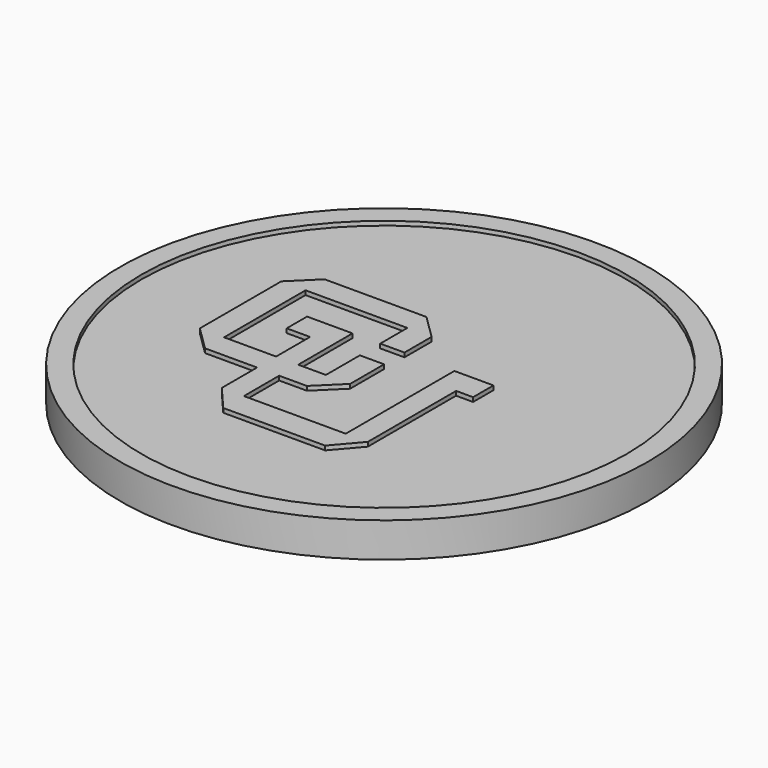
from build123d import *

# Parameters (mm, degrees)
F0_R           = 39.494920522
F1_DEPTH       = 3.81
F2_R           = 39.494920522
F2_R_2         = 36.319920522
F3_DEPTH       = 0.635
F5_TEXT_SIZE   = 15.7882537072
F5_TEXT_SIZE_2 = 16.5979061017
F4_R           = 39.494920522
F4_R_2         = 35.4574187823
F6_DEPTH       = 0.7366


# Not quite as in the source:
# - Text() gives the source's letters only with a copy of the font that has no kerning and outlines rounded to 1/6400 em; it was checked with that copy


with BuildPart() as f1:
    # F0 (on Top) → F1 (new body)
    with BuildSketch(Plane.XY):
        Circle(F0_R)
    extrude(amount=F1_DEPTH)

    # F2 (on face) → F3 (join)
    with BuildSketch(Plane.XY.offset(3.81)):
        Circle(F2_R)
        Circle(F2_R_2, mode=Mode.SUBTRACT)
        Polygon((0, -6.35), (0, 0), (-3.6240225824, 0), (-3.6240225824, -6.35), (-7.7700454983, -6.35), (-7.7700454983, 3.81), (-14.5737715065, 3.81), (-14.5737715065, 0), (-11.0760657117, 0), (-11.0760657117, -6.35), (-18.8640225824, -6.35), (-18.8640225824, 8.89), (-3.6240225824, 8.89), (-3.6240225824, 3.81), (0, 3.81), (0, 8.89), (-3.6240225824, 12.4498961112), (-18.8640225824, 12.4498961112), (-22.4880451648, 8.89), (-22.4880451648, -6.35), (-18.8640225824, -9.9098961112), (-11.0760657117, -9.9098961112), (-11.0760657117, -16.51), (-7.7700454983, -20.3670235089), (7.4699545017, -20.3670235089), (10.7759747151, -16.51), (10.7759747151, 0), (13.3159747151, 0), (13.3159747151, 3.81), (7.4699545017, 3.81), (7.4699545017, -16.51), (-7.7700454983, -16.51), (-7.7700454983, -9.9098961112), (-3.6240225824, -9.9098961112), align=None)
    extrude(amount=F3_DEPTH)

    # F5 (on face) + F4 (on face) → F6 (join)
    with BuildSketch(Plane(origin=(0, 0, 0), x_dir=(1, 0, 0), z_dir=(0, 0, -1))):
        with Locations((-23.0265576392, 13.2621303201)):
            Text('Randy', F5_TEXT_SIZE, font='Open Sans', text_align=(TextAlign.LEFT, TextAlign.BOTTOM))
        with Locations((-26.815738529, -19.0916396677)):
            Text('Guillen', F5_TEXT_SIZE_2, font='Open Sans', text_align=(TextAlign.LEFT, TextAlign.BOTTOM))
    with BuildSketch(Plane(origin=(0, 0, 0), x_dir=(1, 0, 0), z_dir=(0, 0, -1))):
        Circle(F4_R)
        Circle(F4_R_2, mode=Mode.SUBTRACT)
    extrude(amount=F6_DEPTH)


solid = f1.part
